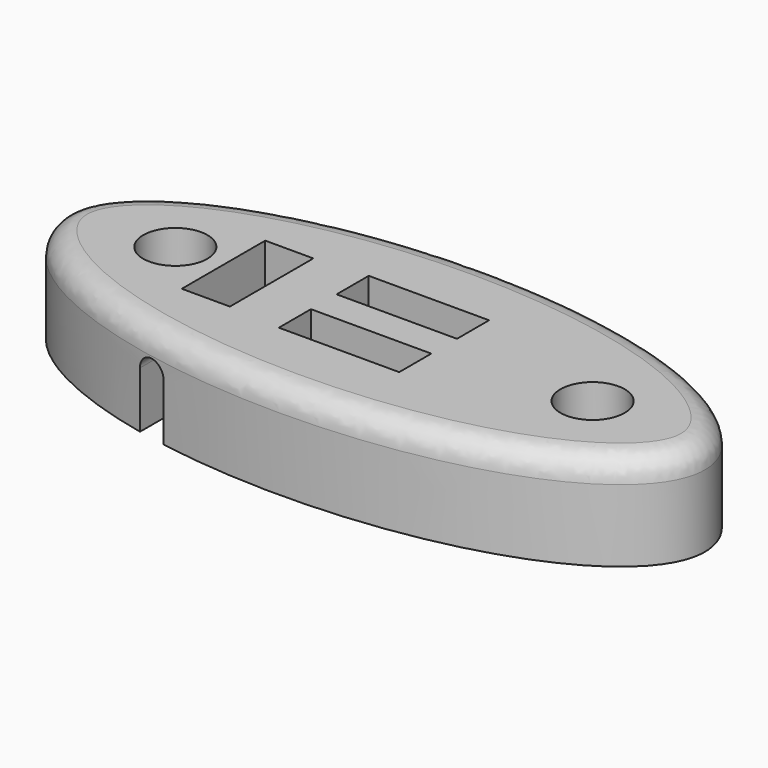
from build123d import *

# Parameters (mm, degrees)
F1_DEPTH = 12
F2_R     = 3
F4_DEPTH = 12.0010001
F5_R     = 4
F6_DEPTH = 53.1
F8_DEPTH = 25


# Not quite as in the source:
# - a feature names something its author has since deleted; it is built from what else it names


with BuildPart() as f1:
    # F0 (on Top) → F1 (new body)
    with BuildSketch(Plane.XY):
        with BuildLine():
            add(Edge.make_bspline(
                [(-40, 0), (-40, -28.5788383249), (20, -14.2894191624), (80, 0), (20, 14.2894191624), (-40, 28.5788383249), (-40, 0)],
                knots=[0, 0, 0, 2.0943951024, 2.0943951024, 4.1887902048, 4.1887902048, 6.2831853072, 6.2831853072, 6.2831853072], degree=2, weights=[1, 0.5, 1, 0.5, 1, 0.5, 1]))
        make_face()
    extrude(amount=F1_DEPTH)

    # F2
    f2_edges = [f1.edges().sort_by_distance(p)[0] for p in [
        (40, -3.8e-05, 12),
    ]]
    fillet(f2_edges, radius=F2_R)

    # F3 (on face) → F4 (cut, through all)
    with BuildSketch(Plane.XY.offset(12)):
        Polygon((7.5, -2), (0, -2), (-7.5, -2), (-7.5, -7), (7.5, -7), align=None)
        Polygon((-7.5, 2), (0, 2), (7.5, 2), (7.5, 7), (-7.5, 7), align=None)
    extrude(amount=-F4_DEPTH, mode=Mode.SUBTRACT)

    # F5 (on face) → F6 (cut)
    with BuildSketch(Plane(origin=(0, 0, 0), x_dir=(1, 0, 0), z_dir=(0, 0, -1))):
        with BuildLine():
            ThreePointArc((-22, 0), (-26, 4), (-30, 0))
            Line((-30, 0), (-26, 0))
            Line((-26, 0), (-22, 0))
        make_face()
        Polygon((-20, 6.5), (-20, 0), (-20, -6.5), (-14, -6.5), (-14, 6.5), align=None)
        with BuildLine():
            Line((-26, 0), (-30, 0))
            ThreePointArc((-30, 0), (-26, -4), (-22, 0))
            Line((-22, 0), (-26, 0))
        make_face()
        with Locations((26, 0)):
            Circle(F5_R)
    extrude(amount=-F6_DEPTH, mode=Mode.SUBTRACT)

    # F7 (on face) → F8 (cut)
    with BuildSketch(Plane(origin=(0, -6.5, 0), x_dir=(-1, 0, 0), z_dir=(0, 1, 0))):
        with BuildLine():
            Line((15.25, 0), (17, 0))
            Line((17, 0), (17, 5.25))
            ThreePointArc((17, 5.25), (15.7625631329, 5.7625631329), (15.25, 7))
            Line((15.25, 7), (15.25, 0))
        make_face()
        with BuildLine():
            Line((17, 5.25), (17, 0))
            Line((17, 0), (18.75, 0))
            Line((18.75, 0), (18.75, 7))
            ThreePointArc((18.75, 7), (18.2374368671, 5.7625631329), (17, 5.25))
        make_face()
        with BuildLine():
            ThreePointArc((15.25, 7), (15.7625631329, 5.7625631329), (17, 5.25))
            ThreePointArc((17, 5.25), (18.2374368671, 5.7625631329), (18.75, 7))
            ThreePointArc((18.75, 7), (17, 8.75), (15.25, 7))
        make_face()
    extrude(amount=-F8_DEPTH, mode=Mode.SUBTRACT)


solid = f1.part
